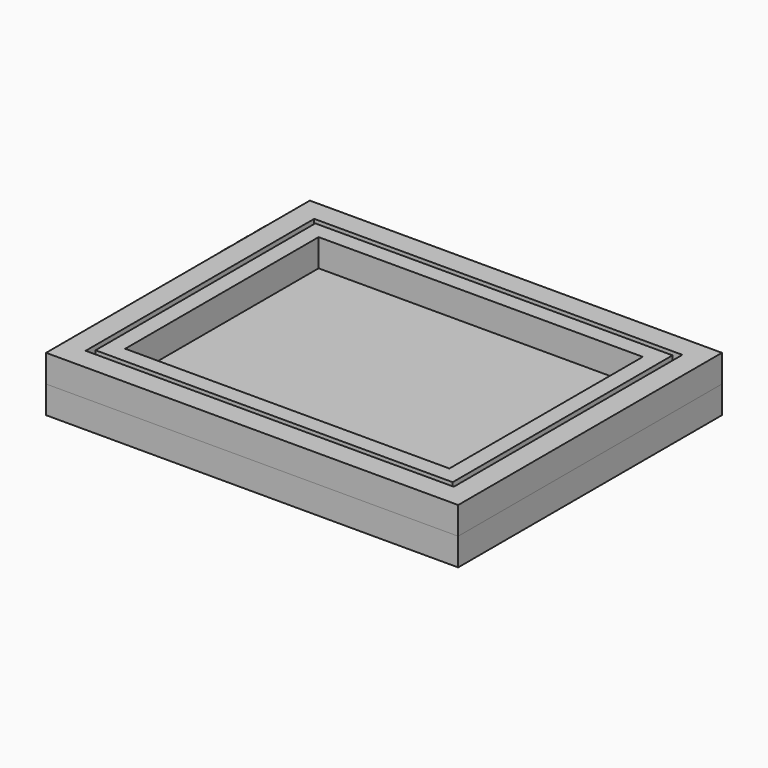
from build123d import *

# Parameters (mm, degrees)
F0_W     = 75
F0_H     = 60
F1_DEPTH = 5
F2_W     = 65
F2_H     = 50
F2_W_2   = 59
F2_H_2   = 44
F3_DEPTH = 5
F4_W     = 75
F4_H     = 60
F4_W_2   = 67
F4_H_2   = 52
F5_DEPTH = 5
F7_DEPTH = 5
F9_DEPTH = 16.0273892857


with BuildPart() as f1:
    # F0 (on Top) → F1 (new body)
    with BuildSketch(Plane.XY):
        Rectangle(F0_W, F0_H)
    extrude(amount=F1_DEPTH)

    # F2 (on face) → F3 (join)
    with BuildSketch(Plane.XY.offset(5)):
        Rectangle(F2_W, F2_H)
        Rectangle(F2_W_2, F2_H_2, mode=Mode.SUBTRACT)
    extrude(amount=F3_DEPTH)

    # F6 (on face) → F7 (join)
    with BuildSketch(Plane(origin=(-37.5, 0, 0), x_dir=(0, -1, 0), z_dir=(-1, 0, 0))):
        Polygon((-21.6927667481, 7.5), (-23.9736107143, 7.5), (-23.9736107143, 1.5), (-13.9736107143, 1.5), (-13.9736107143, 7.5), (-16.2544546806, 7.5), (-16.2544546806, 5), (-17.8331887312, 5), (-17.8331887312, 7.5), (-20.1140326975, 7.5), (-20.1140326975, 5), (-21.6927667481, 5), align=None)
    extrude(amount=F7_DEPTH)

    # F8 (on face) → F9 (cut, through all)
    with BuildSketch(Plane.XZ.offset(-13.9736107143)):
        with BuildLine():
            Line((-42.5, 7.5), (-42.5, 1.5))
            Line((-42.5, 1.5), (-38.4533107281, 1.5))
            add(Edge.make_bspline(
                [(-40, 4.5), (-40.0332466707, 4.2033021988), (-40.0938903512, 3.6621097631), (-39.7141378275, 3.1884036491), (-39.3868051904, 2.8916751674), (-39.0474258601, 2.7075872934), (-38.7521333356, 2.615680849), (-38.4831825305, 2.4911583946), (-38.4607419928, 2.1554776724), (-38.3956996392, 1.9092815912), (-38.4326943281, 1.6464633482), (-38.4533107281, 1.5)],
                knots=[0, 0, 0, 0, 0.1593186871, 0.290605687, 0.4069134712, 0.5144588289, 0.6124296172, 0.7024350291, 0.7986834225, 0.8878102994, 1, 1, 1, 1], degree=3))
            ThreePointArc((-40, 4.5), (-41.5, 6), (-40, 7.5))
            Line((-40, 7.5), (-42.5, 7.5))
        make_face()
    extrude(amount=-F9_DEPTH, mode=Mode.SUBTRACT)


with BuildPart() as f5:
    # F4 (on face) → F5 (new body)
    with BuildSketch(Plane.XY.offset(5)):
        Rectangle(F4_W, F4_H)
        Rectangle(F4_W_2, F4_H_2, mode=Mode.SUBTRACT)
    extrude(amount=F5_DEPTH)


solid = Compound([f1.part, f5.part])
